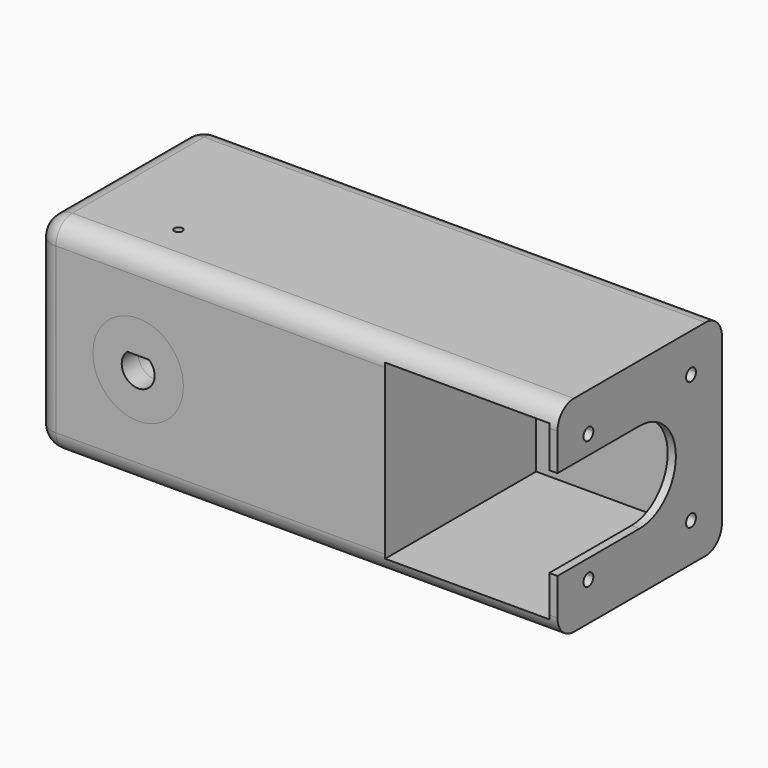
from build123d import *

# Parameters (mm, degrees)
F0_W           = 127
F0_H           = 50
F1_DEPTH       = 50
F3_DEPTH       = 42
F4_R           = 11
F5_DEPTH       = 5
F7_DEPTH       = 15
F8_T2_ANGLE    = 343.7894292622
F9_R           = 5
F12_W          = 40
F12_H          = 42
F13_DEPTH      = 46
F14_R          = 1.6
F15_DEPTH      = 1
F16_R          = 1
F17_DEPTH      = 2
F17_DEPTH_BACK = 1.03
F18_DEPTH      = 25
F19_DEPTH      = 2
F20_DEPTH      = 25
F22_DEPTH      = 8
F23_R          = 2.8130076525
F24_DEPTH      = 3
F25_R          = 0.5
F26_R          = 11
F27_DEPTH      = 5


# Not quite as in the source:
# - a fillet or chamfer that OpenCascade refuses, or shapes differently, is made with other operations: its cross-section is extruded or revolved along the edge and cut away or added


with BuildPart() as f1:
    # F0 (on Front) → F1 (new body)
    with BuildSketch(Plane.XZ):
        Rectangle(F0_W, F0_H)
    extrude(amount=F1_DEPTH)

    # F2 (on face) → F3 (cut)
    with BuildSketch(Plane.YZ.offset(63.5)):
        Polygon((-41.7573593129, 21), (-46, 16.7573593129), (-46, -16.7573593129), (-41.7573593129, -21), (-8.2426406871, -21), (-4, -16.7573593129), (-4, 16.7573593129), (-8.2426406871, 21), align=None)
    extrude(amount=-F3_DEPTH, mode=Mode.SUBTRACT)

    # F4 (on face) → F5 (cut)
    with BuildSketch(Plane.XZ.offset(50)):
        with Locations((-38.5, 0)):
            Circle(F4_R)
    extrude(amount=-F5_DEPTH, mode=Mode.SUBTRACT)

    # F6 (on face) → F7 (cut)
    with BuildSketch(Plane.XZ.offset(45)):
        with BuildLine():
            Line((-37, 2), (-40, 2))
            ThreePointArc((-40, 2), (-38.5, -2.5), (-37, 2))
        make_face()
    extrude(amount=-F7_DEPTH, mode=Mode.SUBTRACT)

    # F8: fillet of radius 0.5 on 1 edges, made by hand

    # F8_s1 → F8_t2 (revolve)
    with BuildSketch(Plane(origin=(-37.7346622942, 0, -5.3739891953), x_dir=(0, 1, 0), z_dir=(0.9900106558, 0, 0.1409925581))):
        with BuildLine():
            ThreePointArc((-30.5, 7.9282134883), (-30.1464466094, 7.7817668789), (-30, 7.4282134883))
            Line((-30, 7.4282134883), (-30, 7.9282134883))
            Line((-30, 7.9282134883), (-30.5, 7.9282134883))
        make_face()
    revolve(axis=Axis((-38.5, -30, 0), (0, -1, 0)), revolution_arc=F8_T2_ANGLE)

    # F9
    f9_edges = [f1.edges().sort_by_distance(p)[0] for p in [
        (0, -50, 25),
        (0, -50, -25),
        (0, 0, 25),
        (0, 0, -25),
        (-63.5, -25, 25),
        (-63.5, -25, -25),
        (-63.5, 0, 0),
        (-63.5, -50, 0),
    ]]
    fillet(f9_edges, radius=F9_R)

    # F12 (on face) → F13 (cut)
    with BuildSketch(Plane.XZ.offset(50)):
        with Locations((41.5, 0)):
            Rectangle(F12_W, F12_H)
    extrude(amount=-F13_DEPTH, mode=Mode.SUBTRACT)

    # F14 (on face) → F15 (cut)
    with BuildSketch(Plane(origin=(0, 0, 0), x_dir=(-1, 0, 0), z_dir=(0, 1, 0))):
        with Locations((-46.0031795697, -4.1205275279)):
            Circle(F14_R)
        with Locations((-22.6282365388, 5.5031795697)):
            Circle(F14_R)
    extrude(amount=-F15_DEPTH, mode=Mode.SUBTRACT)

    # F16 (on face) → F17 (cut, two sides)
    with BuildSketch(Plane(origin=(0, 0, 2), x_dir=(1, 0, 0), z_dir=(0, 0, -1))) as f17_sk:
        Polygon((-36.5, 38.9047005384), (-38.5, 40.0594010768), (-40.5, 38.9047005384), (-40.5, 36.5952994616), (-38.5, 35.4405989232), (-36.5, 36.5952994616), align=None)
        with Locations((-38.5, 37.75)):
            Circle(F16_R, mode=Mode.SUBTRACT)
    extrude(amount=-F17_DEPTH, mode=Mode.SUBTRACT)
    extrude(f17_sk.sketch, amount=F17_DEPTH_BACK, mode=Mode.SUBTRACT)

    # F18 (cut): a face of the model
    f18_faces = [f1.faces().sort_by_distance(p)[0] for p in [
        (-38.5, -37.75, 2),
    ]]
    extrude(f18_faces, amount=-F18_DEPTH, mode=Mode.SUBTRACT)

    # F10 (on face) → F19 (join)
    with BuildSketch(Plane.YZ.offset(63.5)):
        Polygon((-46, 16.7573593129), (-46, -16.7573593129), (-41.7573593129, -21), (-8.2426406871, -21), (-4, -16.7573593129), (-4, 16.7573593129), (-8.2426406871, 21), (-16.9, 21), (-33.1, 21), (-41.7573593129, 21), align=None)
        with BuildLine():
            Line((-10.9, -15.6), (-39.1, -15.6))
            ThreePointArc((-39.1, -15.6), (-41.6606601718, -16.6606601718), (-40.6, -14.1))
            Line((-40.6, -14.1), (-40.6, 14.1))
            ThreePointArc((-40.6, 14.1), (-41.6606601718, 16.6606601718), (-39.1, 15.6))
            Line((-39.1, 15.6), (-10.9, 15.6))
            ThreePointArc((-10.9, 15.6), (-9.4, 17.1), (-7.9, 15.6))
            ThreePointArc((-7.9, 15.6), (-8.3393398282, 14.5393398282), (-9.4, 14.1))
            Line((-9.4, 14.1), (-9.4, -14.1))
            ThreePointArc((-9.4, -14.1), (-8.3393398282, -14.5393398282), (-7.9, -15.6))
            ThreePointArc((-7.9, -15.6), (-9.4, -17.1), (-10.9, -15.6))
        make_face(mode=Mode.SUBTRACT)
        with BuildLine():
            ThreePointArc((-40.6, -14.1), (-39.5393398282, -14.5393398282), (-39.1, -15.6))
            Line((-39.1, -15.6), (-10.9, -15.6))
            ThreePointArc((-10.9, -15.6), (-10.4606601718, -14.5393398282), (-9.4, -14.1))
            Line((-9.4, -14.1), (-9.4, 14.1))
            ThreePointArc((-9.4, 14.1), (-10.4606601718, 14.5393398282), (-10.9, 15.6))
            Line((-10.9, 15.6), (-39.1, 15.6))
            ThreePointArc((-39.1, 15.6), (-39.5393398282, 14.5393398282), (-40.6, 14.1))
            Line((-40.6, 14.1), (-40.6, -14.1))
        make_face()
    extrude(amount=-F19_DEPTH)

    # F11 (on face) → F20 (cut)
    with BuildSketch(Plane.YZ.offset(63.5)):
        with BuildLine():
            Line((-50, -11), (-25, -11))
            ThreePointArc((-25, -11), (-14, 0), (-25, 11))
            Line((-25, 11), (-50, 11))
            Line((-50, 11), (-50, -11))
        make_face()
    extrude(amount=-F20_DEPTH, mode=Mode.SUBTRACT)

    # F21 (on face) → F22 (cut)
    with BuildSketch(Plane.XZ.offset(45)):
        with BuildLine():
            Line((-35.85425, 3.0000011562), (-41.14575, 3.0000011562))
            ThreePointArc((-41.14575, 3.0000011562), (-38.5, -4), (-35.85425, 3.0000011562))
        make_face()
    extrude(amount=-F22_DEPTH, mode=Mode.SUBTRACT)

    # F23 (on face) → F24 (join)
    with BuildSketch(Plane.XZ.offset(37)):
        with Locations((-38.5, 0)):
            Circle(F23_R)
    extrude(amount=-F24_DEPTH)

    # F25
    f25_edges = [f1.edges().sort_by_distance(p)[0] for p in [
        (-38.5, -37, -4),
    ]]
    fillet(f25_edges, radius=F25_R)

    # F26 (on face) → F27 (join, through all)
    with BuildSketch(Plane.XZ.offset(45)):
        with Locations((-38.5, 0)):
            Circle(F26_R)
        with BuildLine():
            ThreePointArc((-35.85425, 3.0000011562), (-38.5, -4), (-41.14575, 3.0000011562))
            Line((-41.14575, 3.0000011562), (-35.85425, 3.0000011562))
        make_face(mode=Mode.SUBTRACT)
    extrude(amount=F27_DEPTH)


solid = f1.part
